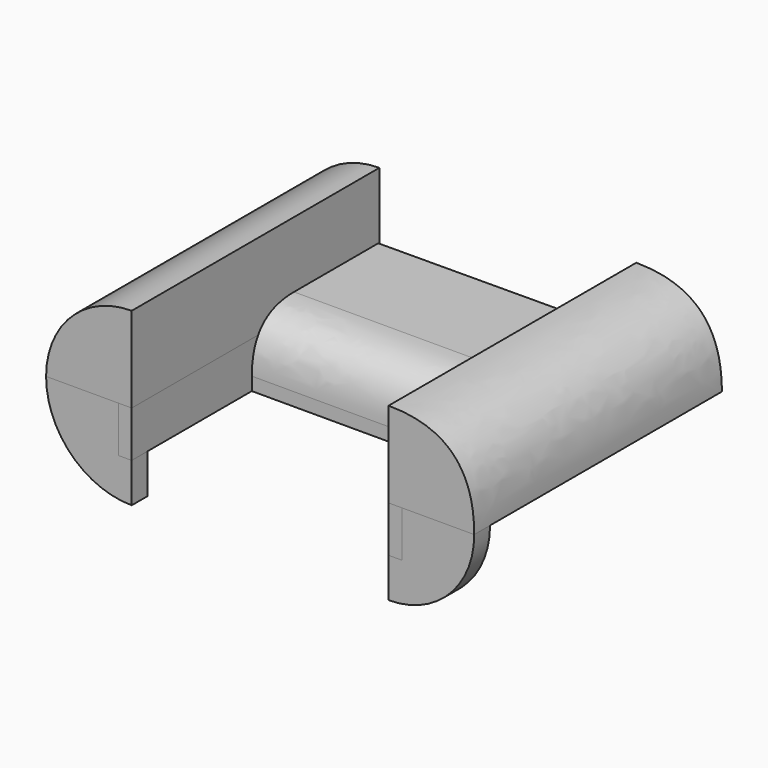
from build123d import *

# Parameters (mm, degrees)
F0_W         = 32.5
F0_H         = 23.5
F1_DEPTH     = 6.5
F2_T1_DEPTH  = 56
F3_R         = 6.49999
F4_DEPTH     = 6.5
F6_DEPTH     = 3.5
F7_W         = 6.5
F7_H         = 6.5
F8_DEPTH     = 1.5
F9_R         = 6.49999
F10_W        = 6.5
F10_H        = 6.5
F11_DEPTH    = 1.5
F12_R        = 6.49999
F13_DEPTH    = 1.5
F14_T1_DEPTH = 39.4996332601
F15_W        = 19.4996332601
F15_H        = 11
F16_DEPTH    = 3.5
F17_W        = 12.4515531301
F17_H        = 3.5
F18_DEPTH    = 1
F19_W        = 12.4432003307
F19_H        = 3.5
F20_DEPTH    = 1


# Not quite as in the source:
# - a fillet or chamfer that OpenCascade refuses, or shapes differently, is made with other operations: its cross-section is extruded or revolved along the edge and cut away or added
# - a fillet or chamfer is up to 0.001 mm smaller than in the source, because OpenCascade refuses the exact size


with BuildPart() as f1:
    # F0 (on Top) → F1 (new body)
    with BuildSketch(Plane.XY):
        Rectangle(F0_W, F0_H)
    extrude(amount=F1_DEPTH)

    # F2: fillet of radius 6.5 on 1 edges, made by hand

    # F2_s2 → F2_t1 (cut)
    with BuildSketch(Plane.XZ.offset(-28)):
        with BuildLine():
            add(Edge.make_bspline(
                [(16.25, 0), (16.25, 6.5), (9.75, 6.5)],
                knots=[0, 0, 0, 1, 1, 1], degree=2, weights=[1, 1, 1]))
            Line((9.75, 6.5), (16.25, 6.5))
            Line((16.25, 6.5), (16.25, 0))
        make_face()
    extrude(amount=F2_T1_DEPTH, mode=Mode.SUBTRACT)

    # F3 (radius 6.5 in the source; OpenCascade refuses exactly that, so slightly less here)
    f3_edges = [f1.edges().sort_by_distance(p)[0] for p in [
        (-16.25, 0, 6.5),
    ]]
    fillet(f3_edges, radius=F3_R)

    # F4 (cut): a face of the model
    f4_faces = [f1.faces().sort_by_distance(p)[0] for p in [
        (-5e-06, 0, 6.5),
    ]]
    extrude(f4_faces, amount=-F4_DEPTH, mode=Mode.SUBTRACT)


with BuildPart() as f6:
    # F5 (on face) → F6 (new body)
    with BuildSketch(Plane(origin=(0, 0, 0), x_dir=(1, 0, 0), z_dir=(0, 0, -1))):
        Polygon((-9.7496332601, 0.3559169248), (-9.7496332601, -11.6440830752), (9.75, -11.75), (9.75, 0.3559169248), align=None)
    extrude(amount=F6_DEPTH)

    # F5 (on face) → F13 (join)
    with BuildSketch(Plane(origin=(0, 0, 0), x_dir=(1, 0, 0), z_dir=(0, 0, -1))):
        Polygon((-9.7496332601, 0.3559169248), (-9.7496332601, -11.6440830752), (9.75, -11.75), (9.75, 0.3559169248), align=None)
    extrude(amount=-F13_DEPTH)

    # F14: fillet of radius 4 on 1 edges, made by hand

    # F14_s2 → F14_t1 (cut)
    with BuildSketch(Plane.YZ.offset(-19.7496332601)):
        with BuildLine():
            add(Edge.make_bspline(
                [(3.6440830752, 1.5), (-0.3559169248, 1.5), (-0.3559169248, -2.5)],
                knots=[0, 0, 0, 1, 1, 1], degree=2, weights=[1, 1, 1]))
            Line((-0.3559169248, -2.5), (-0.3559169248, 1.5))
            Line((-0.3559169248, 1.5), (3.6440830752, 1.5))
        make_face()
    extrude(amount=F14_T1_DEPTH, mode=Mode.SUBTRACT)

    # F15 (on face) → F16 (cut)
    with BuildSketch(Plane(origin=(0, 0, -3.5), x_dir=(1, 0, 0), z_dir=(0, 0, -1))):
        with Locations((0.00018337, -6.25)):
            Rectangle(F15_W, F15_H)
    extrude(amount=-F16_DEPTH, mode=Mode.SUBTRACT)


with BuildPart() as f8:
    # F7 (on face) → F8 (new body)
    with BuildSketch(Plane.XZ.offset(11.75)):
        with Locations((-13, -3.25)):
            Rectangle(F7_W, F7_H)
    extrude(amount=-F8_DEPTH)

    # F9 (radius 6.5 in the source; OpenCascade refuses exactly that, so slightly less here)
    f9_edges = [f8.edges().sort_by_distance(p)[0] for p in [
        (-16.25, -11, -6.5),
    ]]
    fillet(f9_edges, radius=F9_R)


with BuildPart() as f11:
    # F10 (on face) → F11 (new body)
    with BuildSketch(Plane.XZ.offset(11.75)):
        with Locations((13, -3.25)):
            Rectangle(F10_W, F10_H)
    extrude(amount=-F11_DEPTH)

    # F12 (radius 6.5 in the source; OpenCascade refuses exactly that, so slightly less here)
    f12_edges = [f11.edges().sort_by_distance(p)[0] for p in [
        (16.25, -11, -6.5),
    ]]
    fillet(f12_edges, radius=F12_R)


with BuildPart() as f18:
    # F17 (on face) → F18 (new body)
    with BuildSketch(Plane.YZ.offset(-9.75)):
        with Locations((-5.524223435, -1.75)):
            Rectangle(F17_W, F17_H)
    extrude(amount=-F18_DEPTH)


with BuildPart() as f20:
    # F19 (on face) → F20 (new body)
    with BuildSketch(Plane(origin=(9.75, 0, 0), x_dir=(0, -1, 0), z_dir=(-1, 0, 0))):
        with Locations((5.5283998346, -1.75)):
            Rectangle(F19_W, F19_H)
    extrude(amount=-F20_DEPTH)


solid = Compound([f1.part, f6.part, f8.part, f11.part, f18.part, f20.part])
